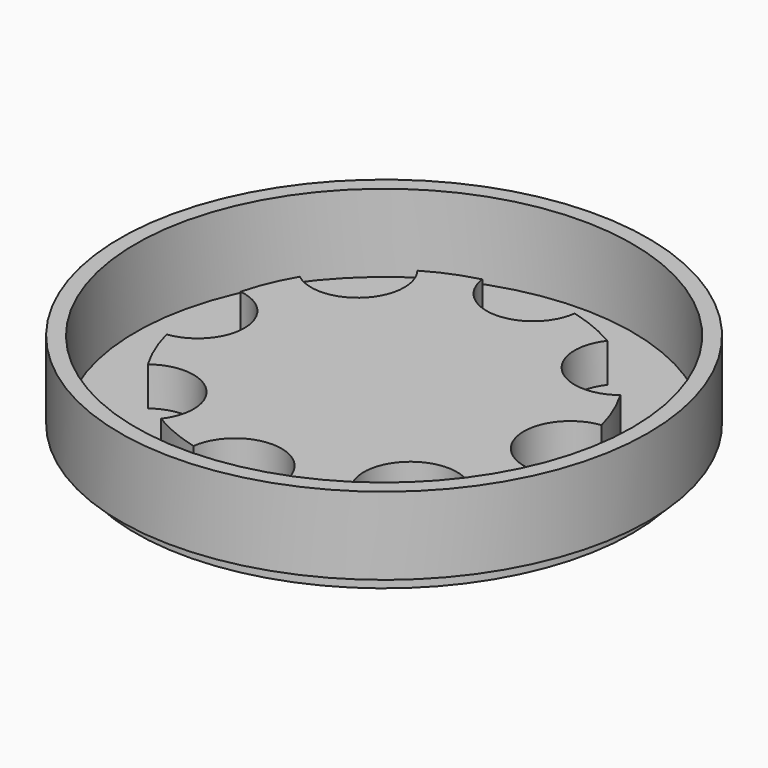
from build123d import *

# Parameters (mm, degrees)
F0_R     = 304.8
F1_DEPTH = 63.5
F3_DEPTH = 480.06
F5_R     = 406.4
F6_DEPTH = 25.4
F5_R_2   = 431.8
F7_DEPTH = 127


with BuildPart() as f1:
    # F0 (on Top) → F1 (new body)
    with BuildSketch(Plane.XY):
        Circle(F0_R)
    extrude(amount=F1_DEPTH)

    # F2 (on face) → F3 (cut)
    with BuildSketch(Plane(origin=(0, 0, 0), x_dir=(1, 0, 0), z_dir=(0, 0, -1))):
        with BuildLine():
            ThreePointArc((75.6023437137, 295.275), (0, 304.8), (-75.6023437137, 295.275))
            ThreePointArc((-75.6023437137, 295.275), (0, 228.6), (75.6023437137, 295.275))
        make_face()
        with BuildLine():
            ThreePointArc((-139.3261469057, 215.5261469057), (-143.4385886978, 240.220760724), (-155.3320249013, 262.2498847284))
            ThreePointArc((-155.3320249013, 262.2498847284), (-215.5261469057, 215.5261469057), (-262.2498847284, 155.3320249013))
            ThreePointArc((-262.2498847284, 155.3320249013), (-182.0142745474, 147.090816768), (-139.3261469057, 215.5261469057))
        make_face()
        with BuildLine():
            ThreePointArc((-228.6, 0), (-247.65, 50.4015624758), (-295.275, 75.6023437137))
            ThreePointArc((-295.275, 75.6023437137), (-304.8, 0), (-295.275, -75.6023437137))
            ThreePointArc((-295.275, -75.6023437137), (-247.65, -50.4015624758), (-228.6, 0))
        make_face()
        with BuildLine():
            ThreePointArc((-139.3261469057, -215.5261469057), (-182.0142745474, -147.090816768), (-262.2498847284, -155.3320249013))
            ThreePointArc((-262.2498847284, -155.3320249013), (-215.5261469057, -215.5261469057), (-155.3320249013, -262.2498847284))
            ThreePointArc((-155.3320249013, -262.2498847284), (-143.4385886978, -240.220760724), (-139.3261469057, -215.5261469057))
        make_face()
        with BuildLine():
            ThreePointArc((75.6023437137, -295.275), (0, -228.6), (-75.6023437137, -295.275))
            ThreePointArc((-75.6023437137, -295.275), (0, -304.8), (75.6023437137, -295.275))
        make_face()
        with BuildLine():
            ThreePointArc((155.3320249013, -262.2498847284), (215.5261469057, -215.5261469057), (262.2498847284, -155.3320249013))
            ThreePointArc((262.2498847284, -155.3320249013), (161.6446101792, -161.6446101792), (155.3320249013, -262.2498847284))
        make_face()
        with BuildLine():
            ThreePointArc((304.8, 0), (302.4093748547, 38.1), (295.275, 75.6023437137))
            ThreePointArc((295.275, 75.6023437137), (228.6, 0), (295.275, -75.6023437137))
            ThreePointArc((295.275, -75.6023437137), (302.4093748547, -38.1), (304.8, 0))
        make_face()
        with BuildLine():
            ThreePointArc((262.2498847284, 155.3320249013), (215.5261469057, 215.5261469057), (155.3320249013, 262.2498847284))
            ThreePointArc((155.3320249013, 262.2498847284), (161.6446101792, 161.6446101792), (262.2498847284, 155.3320249013))
        make_face()
    extrude(amount=-F3_DEPTH, mode=Mode.SUBTRACT)

    # F5 (on face) → F6 (join)
    with BuildSketch(Plane(origin=(0, 0, 0), x_dir=(1, 0, 0), z_dir=(0, 0, -1))):
        Circle(F5_R)
        with BuildLine():
            ThreePointArc((262.2498847284, 155.3320249013), (281.5984815094, 116.6419101849), (295.275, 75.6023437137))
            ThreePointArc((295.275, 75.6023437137), (228.6, 0), (295.275, -75.6023437137))
            ThreePointArc((295.275, -75.6023437137), (281.5984815094, -116.6419101849), (262.2498847284, -155.3320249013))
            ThreePointArc((262.2498847284, -155.3320249013), (161.6446101792, -161.6446101792), (155.3320249013, -262.2498847284))
            ThreePointArc((155.3320249013, -262.2498847284), (116.6419101849, -281.5984815094), (75.6023437137, -295.275))
            ThreePointArc((75.6023437137, -295.275), (0, -228.6), (-75.6023437137, -295.275))
            ThreePointArc((-75.6023437137, -295.275), (-116.6419101849, -281.5984815094), (-155.3320249013, -262.2498847284))
            ThreePointArc((-155.3320249013, -262.2498847284), (-161.6446101792, -161.6446101792), (-262.2498847284, -155.3320249013))
            ThreePointArc((-262.2498847284, -155.3320249013), (-281.5984815094, -116.6419101849), (-295.275, -75.6023437137))
            ThreePointArc((-295.275, -75.6023437137), (-228.6, 0), (-295.275, 75.6023437137))
            ThreePointArc((-295.275, 75.6023437137), (-281.5984815094, 116.6419101849), (-262.2498847284, 155.3320249013))
            ThreePointArc((-262.2498847284, 155.3320249013), (-161.6446101792, 161.6446101792), (-155.3320249013, 262.2498847284))
            ThreePointArc((-155.3320249013, 262.2498847284), (-116.6419101849, 281.5984815094), (-75.6023437137, 295.275))
            ThreePointArc((-75.6023437137, 295.275), (0, 228.6), (75.6023437137, 295.275))
            ThreePointArc((75.6023437137, 295.275), (116.6419101849, 281.5984815094), (155.3320249013, 262.2498847284))
            ThreePointArc((155.3320249013, 262.2498847284), (161.6446101792, 161.6446101792), (262.2498847284, 155.3320249013))
        make_face(mode=Mode.SUBTRACT)
        with BuildLine():
            ThreePointArc((295.275, -75.6023437137), (228.6, 0), (295.275, 75.6023437137))
            ThreePointArc((295.275, 75.6023437137), (281.5984815094, 116.6419101849), (262.2498847284, 155.3320249013))
            ThreePointArc((262.2498847284, 155.3320249013), (161.6446101792, 161.6446101792), (155.3320249013, 262.2498847284))
            ThreePointArc((155.3320249013, 262.2498847284), (116.6419101849, 281.5984815094), (75.6023437137, 295.275))
            ThreePointArc((75.6023437137, 295.275), (0, 228.6), (-75.6023437137, 295.275))
            ThreePointArc((-75.6023437137, 295.275), (-116.6419101849, 281.5984815094), (-155.3320249013, 262.2498847284))
            ThreePointArc((-155.3320249013, 262.2498847284), (-161.6446101792, 161.6446101792), (-262.2498847284, 155.3320249013))
            ThreePointArc((-262.2498847284, 155.3320249013), (-281.5984815094, 116.6419101849), (-295.275, 75.6023437137))
            ThreePointArc((-295.275, 75.6023437137), (-228.6, 0), (-295.275, -75.6023437137))
            ThreePointArc((-295.275, -75.6023437137), (-281.5984815094, -116.6419101849), (-262.2498847284, -155.3320249013))
            ThreePointArc((-262.2498847284, -155.3320249013), (-161.6446101792, -161.6446101792), (-155.3320249013, -262.2498847284))
            ThreePointArc((-155.3320249013, -262.2498847284), (-116.6419101849, -281.5984815094), (-75.6023437137, -295.275))
            ThreePointArc((-75.6023437137, -295.275), (0, -228.6), (75.6023437137, -295.275))
            ThreePointArc((75.6023437137, -295.275), (116.6419101849, -281.5984815094), (155.3320249013, -262.2498847284))
            ThreePointArc((155.3320249013, -262.2498847284), (161.6446101792, -161.6446101792), (262.2498847284, -155.3320249013))
            ThreePointArc((262.2498847284, -155.3320249013), (281.5984815094, -116.6419101849), (295.275, -75.6023437137))
        make_face()
    extrude(amount=F6_DEPTH)


with BuildPart() as f7:
    # F5 (on face) → F7 (new body)
    with BuildSketch(Plane(origin=(0, 0, 0), x_dir=(1, 0, 0), z_dir=(0, 0, -1))):
        Circle(F5_R_2)
        Circle(F5_R, mode=Mode.SUBTRACT)
    extrude(amount=-F7_DEPTH)


solid = Compound([f1.part, f7.part])
